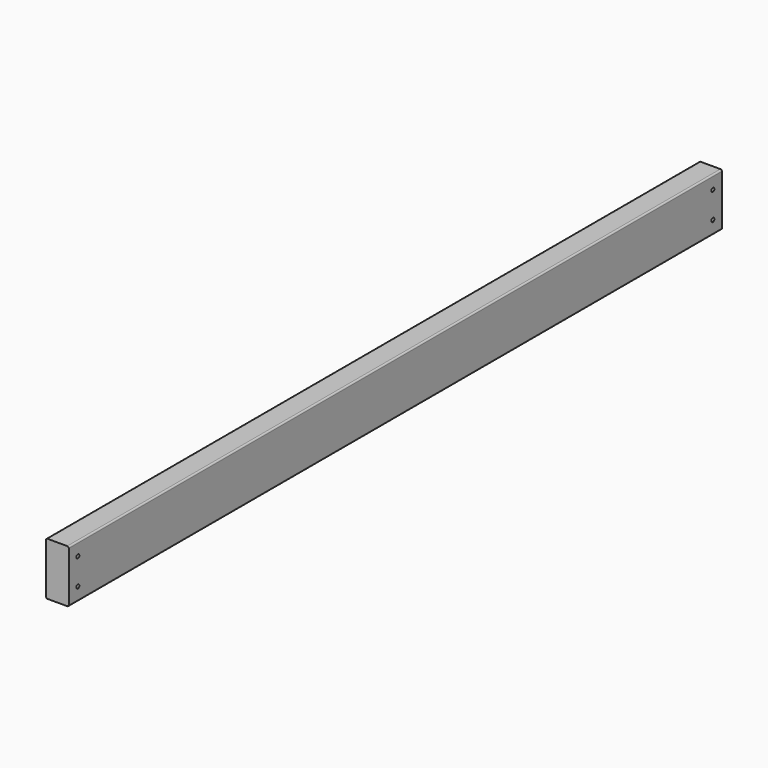
from build123d import *

# Parameters (mm, degrees)
F0_W          = 38.1
F0_H          = 88.9
F1_DEPTH      = 685.8
F1_DEPTH_BACK = 685.8
F2_R          = 3.175
F3_DEPTH      = 12.7
F4_R          = 2.54


# Not quite as in the source:
# - a length typed as a fraction of an inch, garbled in the dataset ("3 / 203.2 mm" for 3/8 in), is restored
# - a pattern or mirror of a feature is missing from the dataset's text; its kind, count and spacing are read off the source's solid


with BuildPart() as f1:
    # F0 (on Front) → F1 (new body, two sides)
    with BuildSketch(Plane.XZ) as f1_sk:
        Rectangle(F0_W, F0_H)
    extrude(amount=F1_DEPTH)
    extrude(f1_sk.sketch, amount=-F1_DEPTH_BACK)

    # F2 (on face) → F3 (cut)
    with BuildSketch(Plane.YZ.offset(19.05)):
        with Locations((-666.75, 22.225)):
            Circle(F2_R)
    f3 = extrude(amount=-F3_DEPTH, mode=Mode.SUBTRACT)

    # F3_copies: F3 across plane
    add(f3.mirror(Plane(origin=(0, 0, 0), x_dir=(0, 0.0333148302, 0.999444907), z_dir=(0, 0.999444907, -0.0333148302))), mode=Mode.SUBTRACT)

    # F3_copies1: F3 across plane
    add(f3.mirror(Plane(origin=(0, 0, 0), x_dir=(-1, 0, 0), z_dir=(0, 0, -1))), mode=Mode.SUBTRACT)

    # F3_copies2: F3 across plane
    add(f3.mirror(Plane.ZX), mode=Mode.SUBTRACT)

    # F4
    f4_edges = [f1.edges().sort_by_distance(p)[0] for p in [
        (19.05, 0, 44.45),
        (-19.05, 0, 44.45),
        (19.05, 0, -44.45),
        (-19.05, 0, -44.45),
    ]]
    fillet(f4_edges, radius=F4_R)


solid = f1.part
